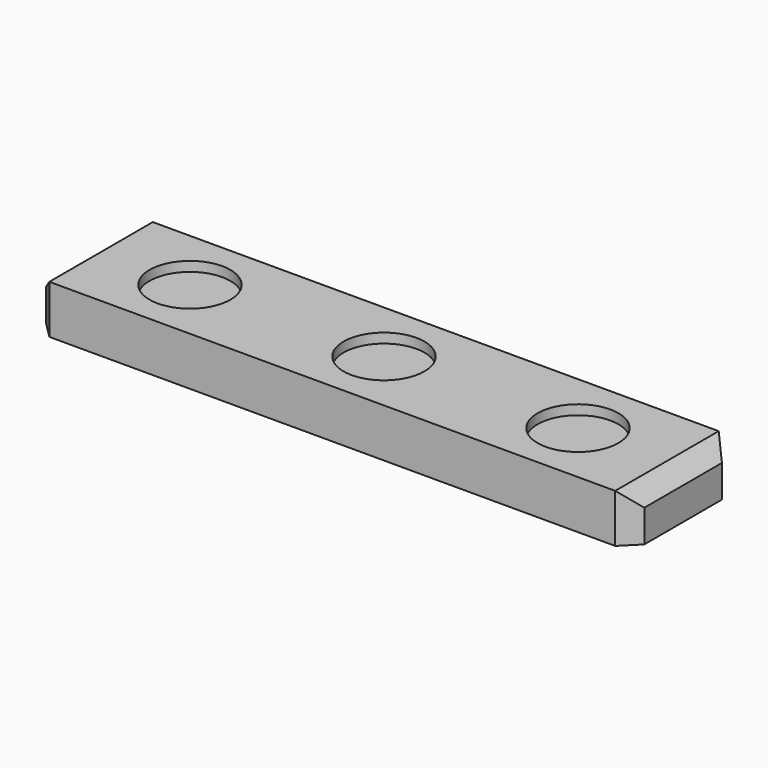
from build123d import *

# Parameters (mm, degrees)
F0_W     = 74
F0_H     = 16
F1_DEPTH = 6
F2_R     = 5
F3_DEPTH = 1.2
F4_SIZE  = 2


# Not quite as in the source:
# - a feature of the source that left no trace in its solid (it failed there, or was rolled back) is left out


with BuildPart() as f1:
    # F0 (on Top) → F1 (new body)
    with BuildSketch(Plane.XY):
        Rectangle(F0_W, F0_H)
    extrude(amount=F1_DEPTH)

    # F2 (on face) → F3 (cut)
    with BuildSketch(Plane.XY.offset(6)):
        with Locations((-24, 0)):
            Circle(F2_R)
        Circle(F2_R)
        with Locations((24, 0)):
            Circle(F2_R)
    extrude(amount=-F3_DEPTH, mode=Mode.SUBTRACT)

    # F4
    f4_edges = [f1.edges().sort_by_distance(p)[0] for p in [
        (-37, 8, 3),
        (-37, -8, 3),
        (37, -8, 3),
        (37, 8, 3),
        (-37, 0, 6),
        (37, 0, 6),
    ]]
    chamfer(f4_edges, length=F4_SIZE)


solid = f1.part
